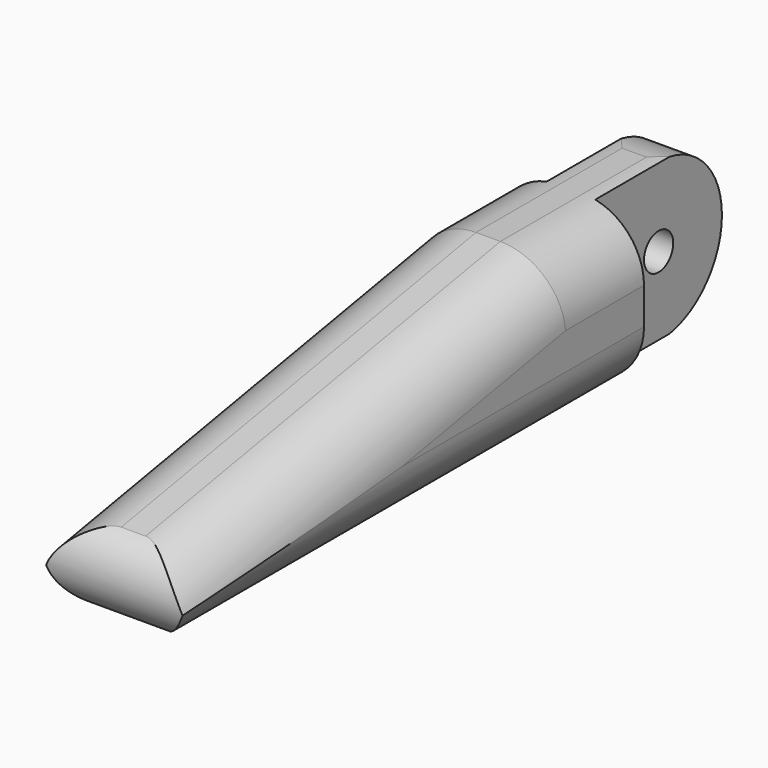
from build123d import *

# Parameters (mm, degrees)
F1_DEPTH     = 12
F2_START     = 4
F0_R         = 1.5
F2_DEPTH     = 4
F3_T1_DEPTH  = 58.5
F3_T3_DEPTH  = 87
F3_T5_DEPTH  = 68.5
F3_T10_ANGLE = 359.64
F3_S11_R     = 5
F3_T12_DEPTH = 7
F3_T16_ANGLE = 359.64
F3_S17_R     = 5
F3_T18_DEPTH = 7
F3_T22_ANGLE = 359.64
F3_S23_R     = 5
F3_T24_DEPTH = 7
F3_T28_ANGLE = 359.64
F3_S29_R     = 5
F3_T30_DEPTH = 7


# Not quite as in the source:
# - a fillet or chamfer that OpenCascade refuses, or shapes differently, is made with other operations: its cross-section is extruded or revolved along the edge and cut away or added


with BuildPart() as f1:
    # F0 (on Right) → F1 (new body)
    with BuildSketch(Plane.YZ):
        with BuildLine():
            Line((-6.5, -6.5), (-6.5, 0))
            Line((-6.5, 0), (-6.5, 6.5))
            Line((-6.5, 6.5), (-15, 6.5))
            Line((-15, 6.5), (-51.4245796132, 0))
            ThreePointArc((-51.4245796132, 0), (-53.3271394273, -3.8230863787), (-50, -6.5))
            Line((-50, -6.5), (-6.5, -6.5))
        make_face()
    extrude(amount=F1_DEPTH)

    # F0 (on Right) → F2 (join)
    with BuildSketch(Plane.YZ.offset(F2_START)):
        with BuildLine():
            ThreePointArc((0, -6.5), (4.5961940777, -4.5961940777), (6.5, 0))
            ThreePointArc((6.5, 0), (4.5961940777, 4.5961940777), (0, 6.5))
            ThreePointArc((0, 6.5), (-4.5961940777, 4.5961940777), (-6.5, 0))
            ThreePointArc((-6.5, 0), (-4.5961940777, -4.5961940777), (0, -6.5))
        make_face()
        Circle(F0_R, mode=Mode.SUBTRACT)
        with BuildLine():
            ThreePointArc((-6.5, 0), (-4.5961940777, 4.5961940777), (0, 6.5))
            Line((0, 6.5), (-6.5, 6.5))
            Line((-6.5, 6.5), (-6.5, 0))
        make_face()
        with BuildLine():
            Line((-6.5, -6.5), (0, -6.5))
            ThreePointArc((0, -6.5), (-4.5961940777, -4.5961940777), (-6.5, 0))
            Line((-6.5, 0), (-6.5, -6.5))
        make_face()
    extrude(amount=F2_DEPTH)

    # F3: fillet of radius 5 on 6 edges, made by hand

    # F3_s2 → F3_t1 (cut)
    with BuildSketch(Plane.XZ.offset(-6)):
        with BuildLine():
            ThreePointArc((12, 1.5), (10.5355339059, 5.0355339059), (7, 6.5))
            Line((7, 6.5), (12, 6.5))
            Line((12, 6.5), (12, 1.5))
        make_face()
        with BuildLine():
            ThreePointArc((0, 1.5), (1.4644660941, 5.0355339059), (5, 6.5))
            Line((5, 6.5), (0, 6.5))
            Line((0, 6.5), (0, 1.5))
        make_face()
    extrude(amount=F3_T1_DEPTH, mode=Mode.SUBTRACT)

    # F3_s4 → F3_t3 (cut)
    with BuildSketch(Plane(origin=(0, 23.5038661081, 4.1942866966), x_dir=(1, 0, 0), z_dir=(0, -0.9844480977, -0.1756756757))):
        with BuildLine():
            ThreePointArc((12, 4.0340477699), (10.5355339059, 7.5695816758), (7, 9.0340477699))
            Line((7, 9.0340477699), (12, 9.0340477699))
            Line((12, 9.0340477699), (12, 4.0340477699))
        make_face()
        with BuildLine():
            ThreePointArc((0, 4.0340477699), (1.4644660941, 7.5695816758), (5, 9.0340477699))
            Line((5, 9.0340477699), (0, 9.0340477699))
            Line((0, 9.0340477699), (0, 4.0340477699))
        make_face()
    extrude(amount=F3_T3_DEPTH, mode=Mode.SUBTRACT)

    # F3_s6 → F3_t5 (cut)
    with BuildSketch(Plane.XZ.offset(-6)):
        with BuildLine():
            ThreePointArc((5, -6.5), (1.4644660941, -5.0355339059), (0, -1.5))
            Line((0, -1.5), (0, -6.5))
            Line((0, -6.5), (5, -6.5))
        make_face()
        with BuildLine():
            ThreePointArc((7, -6.5), (10.5355339059, -5.0355339059), (12, -1.5))
            Line((12, -1.5), (12, -6.5))
            Line((12, -6.5), (7, -6.5))
        make_face()
    extrude(amount=F3_T5_DEPTH, mode=Mode.SUBTRACT)


with BuildPart() as f3_tool8:
    # F3_s9 → F3_t10 (revolve)
    with BuildSketch(Plane(origin=(0, -50.0174650791, -0.3142731374), x_dir=(1, 0, 0), z_dir=(0, -0.9999802609, -0.006283144))):
        with BuildLine():
            ThreePointArc((7, -6.185781731), (9.9180943161, -5.2459203447), (11.7391469644, -2.779671956))
            Line((11.7391469644, -2.779671956), (12, -2.779671956))
            Line((12, -2.779671956), (12, -6.185781731))
            Line((12, -6.185781731), (7, -6.185781731))
        make_face()
    revolve(axis=Axis((12, -50, -3.093890225), (1, 0, 0)), revolution_arc=F3_T10_ANGLE)

    # F3_s11 → F3_t12 (cut, symmetric)
    with BuildSketch(Plane(origin=(0, -49.0255152632, -8.7486486486), x_dir=(1, 0, 0), z_dir=(0, 0.9844480977, 0.1756756757))):
        with Locations((7, -4.0340477699)):
            Circle(F3_S11_R)
    extrude(amount=F3_T12_DEPTH, both=True, mode=Mode.SUBTRACT)


with BuildPart() as f1_1:
    add(f1.part)

    # F3_t7: cut F3_tool8
    add(f3_tool8.part, mode=Mode.SUBTRACT)


with BuildPart() as f3_tool14:
    # F3_s15 → F3_t16 (revolve)
    with BuildSketch(Plane(origin=(0, -50.0174650791, -0.3142731374), x_dir=(1, 0, 0), z_dir=(0, -0.9999802609, -0.006283144))):
        with BuildLine():
            ThreePointArc((7, -6.185781731), (9.9180943161, -5.2459203447), (11.7391469644, -2.779671956))
            Line((11.7391469644, -2.779671956), (12, -2.779671956))
            Line((12, -2.779671956), (12, -6.185781731))
            Line((12, -6.185781731), (7, -6.185781731))
        make_face()
    revolve(axis=Axis((12, -50, -3.093890225), (1, 0, 0)), revolution_arc=F3_T16_ANGLE)

    # F3_s17 → F3_t18 (cut, symmetric)
    with BuildSketch(Plane.XZ.offset(50)):
        with Locations((7, -1.5)):
            Circle(F3_S17_R)
    extrude(amount=F3_T18_DEPTH, both=True, mode=Mode.SUBTRACT)


with BuildPart() as f1_2:
    add(f1_1.part)

    # F3_t13: cut F3_tool14
    add(f3_tool14.part, mode=Mode.SUBTRACT)


with BuildPart() as f3_tool20:
    # F3_s21 → F3_t22 (revolve)
    with BuildSketch(Plane(origin=(0, -50.0174650791, -0.3142731374), x_dir=(1, 0, 0), z_dir=(0, -0.9999802609, -0.006283144))):
        with BuildLine():
            ThreePointArc((5, -6.185781731), (2.0819056839, -5.2459203447), (0.2608530356, -2.779671956))
            Line((0.2608530356, -2.779671956), (0, -2.779671956))
            Line((0, -2.779671956), (0, -6.185781731))
            Line((0, -6.185781731), (5, -6.185781731))
        make_face()
    revolve(axis=Axis((0, -50, -3.093890225), (1, 0, 0)), revolution_arc=F3_T22_ANGLE)

    # F3_s23 → F3_t24 (cut, symmetric)
    with BuildSketch(Plane(origin=(0, -49.0255152632, -8.7486486486), x_dir=(1, 0, 0), z_dir=(0, 0.9844480977, 0.1756756757))):
        with Locations((5, -4.0340477699)):
            Circle(F3_S23_R)
    extrude(amount=F3_T24_DEPTH, both=True, mode=Mode.SUBTRACT)


with BuildPart() as f1_3:
    add(f1_2.part)

    # F3_t19: cut F3_tool20
    add(f3_tool20.part, mode=Mode.SUBTRACT)


with BuildPart() as f3_tool26:
    # F3_s27 → F3_t28 (revolve)
    with BuildSketch(Plane(origin=(0, -50.0174650791, -0.3142731374), x_dir=(1, 0, 0), z_dir=(0, -0.9999802609, -0.006283144))):
        with BuildLine():
            ThreePointArc((5, -6.185781731), (2.0819056839, -5.2459203447), (0.2608530356, -2.779671956))
            Line((0.2608530356, -2.779671956), (0, -2.779671956))
            Line((0, -2.779671956), (0, -6.185781731))
            Line((0, -6.185781731), (5, -6.185781731))
        make_face()
    revolve(axis=Axis((0, -50, -3.093890225), (1, 0, 0)), revolution_arc=F3_T28_ANGLE)

    # F3_s29 → F3_t30 (cut, symmetric)
    with BuildSketch(Plane.XZ.offset(50)):
        with Locations((5, -1.5)):
            Circle(F3_S29_R)
    extrude(amount=F3_T30_DEPTH, both=True, mode=Mode.SUBTRACT)


with BuildPart() as f1_4:
    add(f1_3.part)

    # F3_t25: cut F3_tool26
    add(f3_tool26.part, mode=Mode.SUBTRACT)


solid = f1_4.part
